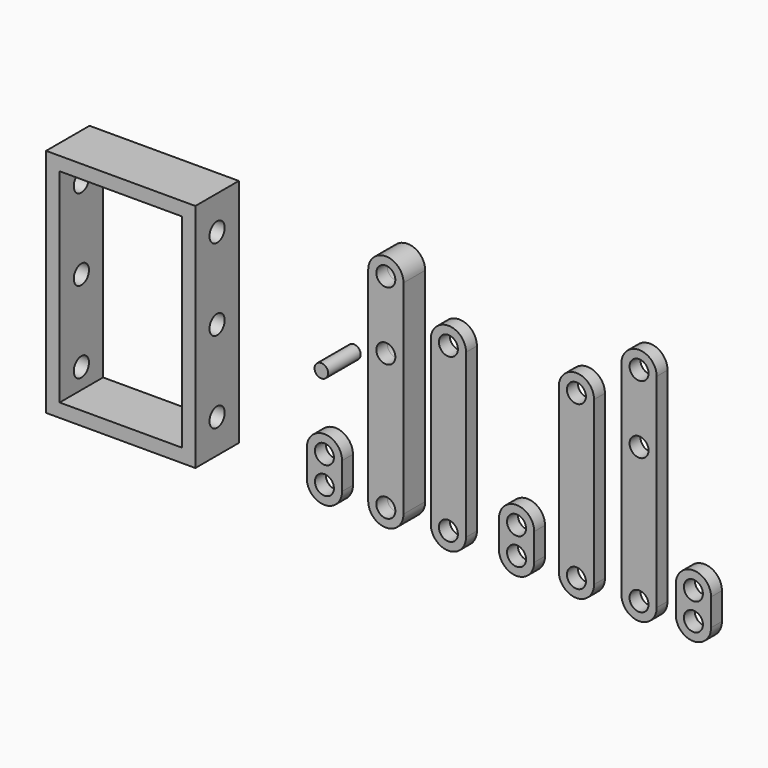
from build123d import *

# Parameters (mm, degrees)
F1_R     = 3.5
F2_DEPTH = 5
F3_R     = 2.5
F4_DEPTH = 15
F5_W     = 55
F5_H     = 85
F5_W_2   = 45
F5_H_2   = 75
F6_DEPTH = 20
F7_R     = 3.5
F8_DEPTH = 55


with BuildPart() as f2:
    # F1 (on Front) → F2 (new body)
    with BuildSketch(Plane.XZ):
        with BuildLine():
            Line((3.3614133894, 10), (3.3614133894, 0))
            ThreePointArc((3.3614133894, 0), (9.8614133894, -6.5), (16.3614133894, 0))
            Line((16.3614133894, 0), (16.3614133894, 10))
            ThreePointArc((16.3614133894, 10), (9.8614133894, 16.5), (3.3614133894, 10))
        make_face()
        with Locations((9.8614133894, 0)):
            Circle(F1_R, mode=Mode.SUBTRACT)
        with Locations((9.8614133894, 10)):
            Circle(F1_R, mode=Mode.SUBTRACT)
    extrude(amount=F2_DEPTH)


with BuildPart() as f2b:
    # F1 (on Front) → F2, piece 2 (new body)
    with BuildSketch(Plane.XZ):
        with BuildLine():
            Line((25.9815175587, 75), (25.9815175587, 0))
            ThreePointArc((25.9815175587, 0), (32.4815175587, -6.5), (38.9815175587, 0))
            Line((38.9815175587, 0), (38.9815175587, 75))
            ThreePointArc((38.9815175587, 75), (32.4815175587, 81.5), (25.9815175587, 75))
        make_face()
        with Locations((32.4815175587, 0)):
            Circle(F1_R, mode=Mode.SUBTRACT)
        with Locations((32.4815175587, 50)):
            Circle(F1_R, mode=Mode.SUBTRACT)
        with Locations((32.4815175587, 75)):
            Circle(F1_R, mode=Mode.SUBTRACT)
    extrude(amount=F2_DEPTH)

    # F9: F2b across plane


with BuildPart() as f2c:
    # F1 (on Front) → F2, piece 3 (new body)
    with BuildSketch(Plane.XZ):
        with BuildLine():
            Line((49.0297546089, 60), (49.0297546089, 0))
            ThreePointArc((49.0297546089, 0), (55.5297546089, -6.5), (62.0297546089, 0))
            Line((62.0297546089, 0), (62.0297546089, 60))
            ThreePointArc((62.0297546089, 60), (55.5297546089, 66.5), (49.0297546089, 60))
        make_face()
        with Locations((55.5297546089, 0)):
            Circle(F1_R, mode=Mode.SUBTRACT)
        with Locations((55.5297546089, 60)):
            Circle(F1_R, mode=Mode.SUBTRACT)
    extrude(amount=F2_DEPTH)


with BuildPart() as f2d:
    # F1 (on Front) → F2, piece 4 (new body)
    with BuildSketch(Plane.XZ):
        with BuildLine():
            Line((74.1323289871, 10), (74.1323289871, 0))
            ThreePointArc((74.1323289871, 0), (80.6323289871, -6.5), (87.1323289871, 0))
            Line((87.1323289871, 0), (87.1323289871, 10))
            ThreePointArc((87.1323289871, 10), (80.6323289871, 16.5), (74.1323289871, 10))
        make_face()
        with Locations((80.6323289871, 0)):
            Circle(F1_R, mode=Mode.SUBTRACT)
        with Locations((80.6323289871, 10)):
            Circle(F1_R, mode=Mode.SUBTRACT)
    extrude(amount=F2_DEPTH)


with BuildPart() as f2e:
    # F1 (on Front) → F2, piece 5 (new body)
    with BuildSketch(Plane.XZ):
        with BuildLine():
            Line((96.1921570301, 60), (96.1921570301, 0))
            ThreePointArc((96.1921570301, 0), (102.6921570301, -6.5), (109.1921570301, 0))
            Line((109.1921570301, 0), (109.1921570301, 60))
            ThreePointArc((109.1921570301, 60), (102.6921570301, 66.5), (96.1921570301, 60))
        make_face()
        with Locations((102.6921570301, 0)):
            Circle(F1_R, mode=Mode.SUBTRACT)
        with Locations((102.6921570301, 60)):
            Circle(F1_R, mode=Mode.SUBTRACT)
    extrude(amount=F2_DEPTH)


with BuildPart() as f2f:
    # F1 (on Front) → F2, piece 6 (new body)
    with BuildSketch(Plane.XZ):
        with BuildLine():
            Line((119.2662475109, 75), (119.2662475109, 0))
            ThreePointArc((119.2662475109, 0), (125.7662475109, -6.5), (132.2662475109, 0))
            Line((132.2662475109, 0), (132.2662475109, 75))
            ThreePointArc((132.2662475109, 75), (125.7662475109, 81.5), (119.2662475109, 75))
        make_face()
        with Locations((125.7662475109, 0)):
            Circle(F1_R, mode=Mode.SUBTRACT)
        with Locations((125.7662475109, 50)):
            Circle(F1_R, mode=Mode.SUBTRACT)
        with Locations((125.7662475109, 75)):
            Circle(F1_R, mode=Mode.SUBTRACT)
    extrude(amount=F2_DEPTH)


with BuildPart() as f2g:
    # F1 (on Front) → F2, piece 7 (new body)
    with BuildSketch(Plane.XZ):
        with BuildLine():
            Line((139.2975953817, 10), (139.2975953817, 0))
            ThreePointArc((139.2975953817, 0), (145.7975953817, -6.5), (152.2975953817, 0))
            Line((152.2975953817, 0), (152.2975953817, 10))
            ThreePointArc((152.2975953817, 10), (145.7975953817, 16.5), (139.2975953817, 10))
        make_face()
        with Locations((145.7975953817, 0)):
            Circle(F1_R, mode=Mode.SUBTRACT)
        with Locations((145.7975953817, 10)):
            Circle(F1_R, mode=Mode.SUBTRACT)
    extrude(amount=F2_DEPTH)


with BuildPart() as f4:
    # F3 (on Front) → F4 (new body)
    with BuildSketch(Plane.XZ):
        with Locations((16.7107470334, 43.3092899621)):
            Circle(F3_R)
    extrude(amount=F4_DEPTH)


with BuildPart() as f6:
    # F5 (on Front) → F6 (new body)
    with BuildSketch(Plane.XZ):
        with Locations((-53.1880603731, 42.5)):
            Rectangle(F5_W, F5_H)
        with Locations((-53.1880603731, 42.5)):
            Rectangle(F5_W_2, F5_H_2, mode=Mode.SUBTRACT)
    extrude(amount=F6_DEPTH)

    # F7 (on face) → F8 (cut, through all)
    with BuildSketch(Plane(origin=(-80.6880603731, 0, 0), x_dir=(0, -1, 0), z_dir=(-1, 0, 0))):
        with Locations((10, 72.5)):
            Circle(F7_R)
        with Locations((10, 42.5)):
            Circle(F7_R)
        with Locations((10, 12.5)):
            Circle(F7_R)
    extrude(amount=-F8_DEPTH, mode=Mode.SUBTRACT)


with BuildPart() as f2b_1:
    add(f2b.part)
    add(f2b.part.mirror(Plane.XZ))


solid = Compound([f2.part, f2c.part, f2d.part, f2e.part, f2f.part, f2g.part, f4.part, f6.part, f2b_1.part])
